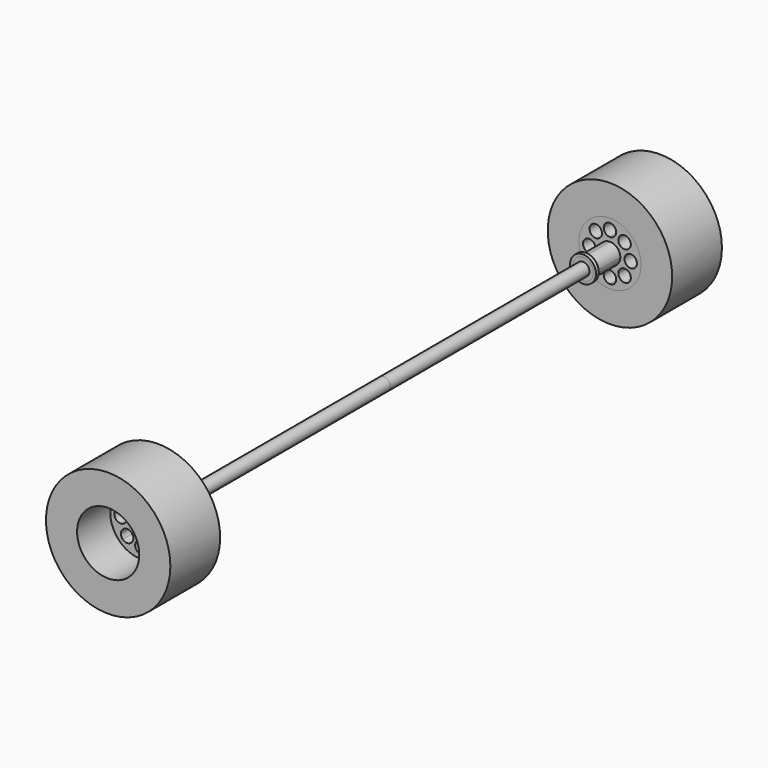
from build123d import *

# Parameters (mm, degrees)
F0_R     = 19.05
F0_R_2   = 9.525
F1_DEPTH = 19.05
F2_DEPTH = 6.35
F4_DEPTH = 10.31875
F3_R     = 1.905
F5_DEPTH = 6.35
F6_R     = 3.96875
F6_R_2   = 3.175
F7_DEPTH = 1.5875
F8_SIZE  = 0.508
F6_R_3   = 1.984375
F9_DEPTH = 76.2


with BuildPart() as f1:
    # F0 (on Front) → F1 (new body)
    with BuildSketch(Plane.XZ):
        Circle(F0_R)
        Circle(F0_R_2, mode=Mode.SUBTRACT)
    extrude(amount=F1_DEPTH)


with BuildPart() as f2:
    # F0 (on Front) → F2 (new body)
    with BuildSketch(Plane.XZ):
        Circle(F0_R_2)
    extrude(amount=F2_DEPTH)

    # F3 (on face) → F4 (join)
    with BuildSketch(Plane(origin=(0, 0, 0), x_dir=(-1, 0, 0), z_dir=(0, 1, 0))):
        with BuildLine():
            Line((3.175, 0), (0, 0))
            Line((0, 0), (0, -3.175))
            ThreePointArc((0, -3.175), (1.1049251721, -2.9765357992), (2.0717161135, -2.4059545601))
            ThreePointArc((2.0717161135, -2.4059545601), (2.88602873, -1.3234285662), (3.175, 0))
        make_face()
        with BuildLine():
            ThreePointArc((3.175, 0), (2.2450640303, 2.2450640303), (0, 3.175))
            Line((0, 3.175), (0, 0))
            Line((0, 0), (3.175, 0))
        make_face()
        with BuildLine():
            ThreePointArc((0, 3.175), (-2.2450640303, 2.2450640303), (-3.175, 0))
            Line((-3.175, 0), (0, 0))
            Line((0, 0), (0, 3.175))
        make_face()
        with BuildLine():
            Line((0, 0), (-2.2450640303, -2.2450640303))
            ThreePointArc((-2.2450640303, -2.2450640303), (-1.2150198978, -2.9333175157), (0, -3.175))
            Line((0, -3.175), (0, 0))
        make_face()
        with BuildLine():
            Line((0, 0), (-3.175, 0))
            ThreePointArc((-3.175, 0), (-2.9333175157, -1.2150198978), (-2.2450640303, -2.2450640303))
            Line((-2.2450640303, -2.2450640303), (0, 0))
        make_face()
    extrude(amount=F4_DEPTH)

    # F3 (on face) → F5 (cut)
    with BuildSketch(Plane(origin=(0, 0, 0), x_dir=(-1, 0, 0), z_dir=(0, 1, 0))):
        with Locations((4.3380962214, 4.6346866725)):
            Circle(F3_R)
        with BuildLine():
            Line((8.255, 0), (4.445, 0))
            ThreePointArc((4.445, 0), (6.35, -1.905), (8.255, 0))
        make_face()
        with BuildLine():
            ThreePointArc((8.255, 0), (6.35, 1.905), (4.445, 0))
            Line((4.445, 0), (8.255, 0))
        make_face()
        with BuildLine():
            ThreePointArc((6.2430962214, -4.6346866725), (5.0597317217, -2.8716588211), (2.9798235656, -3.2989769763))
            Line((2.9798235656, -3.2989769763), (5.6963688772, -5.9703963686))
            ThreePointArc((5.6963688772, -5.9703963686), (6.1011240727, -5.3563221728), (6.2430962214, -4.6346866725))
        make_face()
        with BuildLine():
            Line((5.6963688772, -5.9703963686), (2.9798235656, -3.2989769763))
            ThreePointArc((2.9798235656, -3.2989769763), (3.0023865252, -5.9929593283), (5.6963688772, -5.9703963686))
        make_face()
        with BuildLine():
            Line((0, -8.255), (0, -4.445))
            ThreePointArc((0, -4.445), (-1.905, -6.35), (0, -8.255))
        make_face()
        with BuildLine():
            ThreePointArc((1.905, -6.35), (1.3470384182, -5.0029615818), (0, -4.445))
            Line((0, -4.445), (0, -8.255))
            ThreePointArc((0, -8.255), (1.3470384182, -7.6970384182), (1.905, -6.35))
        make_face()
        with BuildLine():
            Line((-5.8371664787, -5.8371664787), (-3.1430896424, -3.1430896424))
            ThreePointArc((-3.1430896424, -3.1430896424), (-5.8371664787, -3.1430896424), (-5.8371664787, -5.8371664787))
        make_face()
        with BuildLine():
            ThreePointArc((-2.5851280605, -4.4901280605), (-2.7301375511, -3.7611161219), (-3.1430896424, -3.1430896424))
            Line((-3.1430896424, -3.1430896424), (-5.8371664787, -5.8371664787))
            ThreePointArc((-5.8371664787, -5.8371664787), (-3.7611161219, -6.25011857), (-2.5851280605, -4.4901280605))
        make_face()
        with BuildLine():
            Line((-8.255, 0), (-4.445, 0))
            ThreePointArc((-4.445, 0), (-6.35, 1.905), (-8.255, 0))
        make_face()
        with BuildLine():
            ThreePointArc((-8.255, 0), (-6.35, -1.905), (-4.445, 0))
            Line((-4.445, 0), (-8.255, 0))
        make_face()
        with Locations((-4.4901280605, 4.4901280605)):
            Circle(F3_R)
        with BuildLine():
            ThreePointArc((0, 8.255), (-1.905, 6.35), (0, 4.445))
            Line((0, 4.445), (0, 8.255))
        make_face()
        with BuildLine():
            Line((0, 8.255), (0, 4.445))
            ThreePointArc((0, 4.445), (1.3470384182, 5.0029615818), (1.905, 6.35))
            ThreePointArc((1.905, 6.35), (1.3470384182, 7.6970384182), (0, 8.255))
        make_face()
    extrude(amount=-F5_DEPTH, mode=Mode.SUBTRACT)

    # F6 (on face) → F9 (join)
    with BuildSketch(Plane(origin=(0, 10.31875, 0), x_dir=(-1, 0, 0), z_dir=(0, 1, 0))):
        Circle(F6_R_3)
    extrude(amount=F9_DEPTH)


with BuildPart() as f7:
    # F6 (on face) → F7 (new body)
    with BuildSketch(Plane(origin=(0, 10.31875, 0), x_dir=(-1, 0, 0), z_dir=(0, 1, 0))):
        Circle(F6_R)
        Circle(F6_R_2, mode=Mode.SUBTRACT)
    extrude(amount=-F7_DEPTH)

    # F8
    f8_edges = [f7.edges().sort_by_distance(p)[0] for p in [
        (3.96875, 8.73125, 0),
    ]]
    chamfer(f8_edges, length=F8_SIZE)


with BuildPart() as f10_1:
    # F10: instance of F1
    add(f1.part.mirror(Plane(origin=(0, 86.51875, 0), x_dir=(-1, 0, 0), z_dir=(0, 1, 0))))


with BuildPart() as f10_2:
    # F10: instance of F2
    add(f2.part.mirror(Plane(origin=(0, 86.51875, 0), x_dir=(-1, 0, 0), z_dir=(0, 1, 0))))


with BuildPart() as f10_3:
    # F10: instance of F7
    add(f7.part.mirror(Plane(origin=(0, 86.51875, 0), x_dir=(-1, 0, 0), z_dir=(0, 1, 0))))


solid = Compound([f1.part, f2.part, f7.part, f10_1.part, f10_2.part, f10_3.part])
